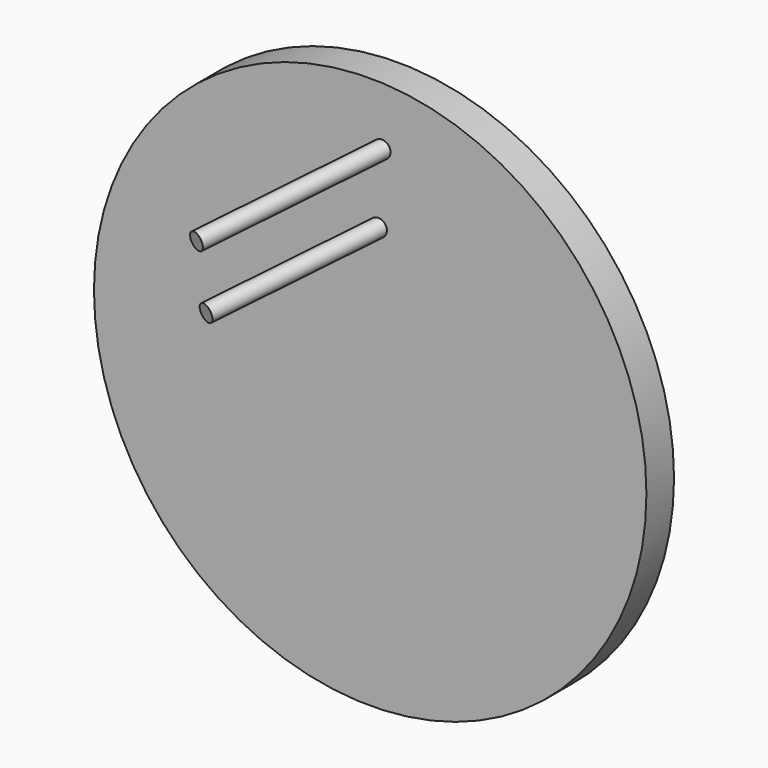
from build123d import *

# Parameters (mm, degrees)
F0_R     = 50.8
F1_DEPTH = 6.35
F5_R     = 1.5875


# Not quite as in the source:
# - a length typed as a fraction of an inch, garbled in the dataset ("3 / 203.2 mm" for 3/8 in), is restored


with BuildPart() as f1:
    # F0 (on Front) → F1 (new body)
    with BuildSketch(Plane.XZ):
        Circle(F0_R)
    extrude(amount=-F1_DEPTH)


with BuildPart() as f6:
    # F5 (on offset) → F6 (new body, up to the next surface of F1)
    with BuildSketch(Plane(origin=(-7.3157607037, -23.9541129475, -4.2237564116), x_dir=(-0.9576237697, 0.2836463724, 0.0500145084), z_dir=(0.2880220749, 0.9430753129, 0.1662896225))):
        with Locations((0, 26.6455678842)):
            Circle(F5_R)
    extrude(until=Until.NEXT, target=f1.part)


with BuildPart() as f6b:
    # F5 (on offset) → F6, piece 2 (new body, up to the next surface of F1)
    with BuildSketch(Plane(origin=(-7.3157607037, -23.9541129475, -4.2237564116), x_dir=(-0.9576237697, 0.2836463724, 0.0500145084), z_dir=(0.2880220749, 0.9430753129, 0.1662896225))):
        with Locations((0, 39.3455678842)):
            Circle(F5_R)
    extrude(until=Until.NEXT, target=f1.part)


solid = Compound([f1.part, f6.part, f6b.part])
